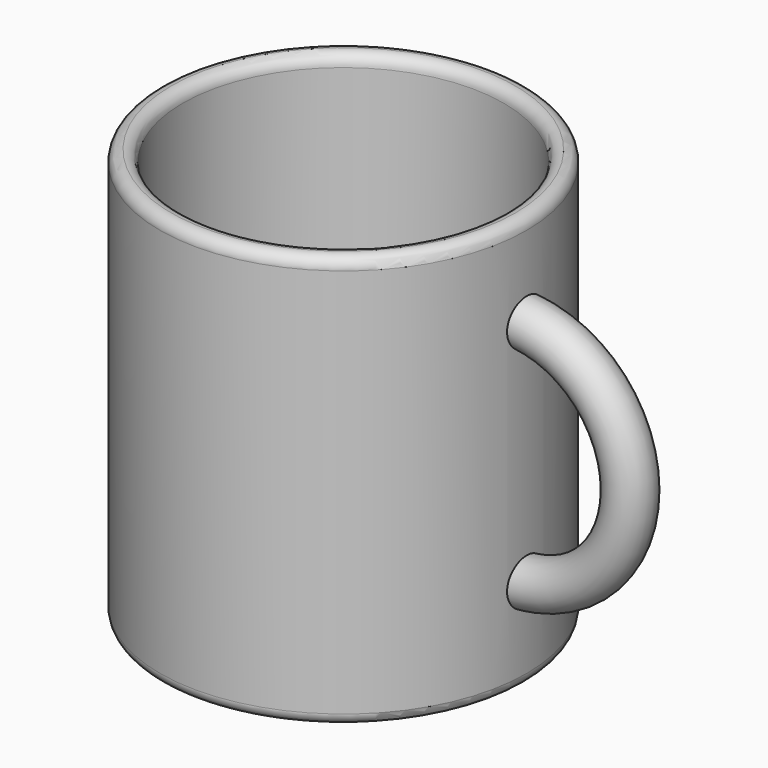
from build123d import *

# Parameters (mm, degrees)
F0_R         = 40
F1_DEPTH     = 90
F2_T         = -5
F4_R         = 5
F5_ANGLE     = 180
F6_R         = 2.49999
F7_TEXT_SIZE = 17.4750366973
F8_DEPTH     = 2.5


# Not quite as in the source:
# - a fillet or chamfer is up to 0.001 mm smaller than in the source, because OpenCascade refuses the exact size
# - Text() gives the source's letters only with a copy of the font that has no kerning and outlines rounded to 1/6400 em; it was checked with that copy


with BuildPart() as f1:
    # F0 (on Top) → F1 (new body)
    with BuildSketch(Plane.XY):
        Circle(F0_R)
    extrude(amount=F1_DEPTH)

    # F2
    f2_openings = [f1.faces().sort_by_distance(p)[0] for p in [
        (0, 0, 90),
    ]]
    offset(amount=F2_T, openings=f2_openings)

    # F4 (on offset) → F5 (revolve)
    with BuildSketch(Plane.YZ.offset(37.5)):
        with Locations((0, 70)):
            Circle(F4_R)
    revolve(axis=Axis((37.5, 15.199537389, 45), (0, 1, 0)), revolution_arc=F5_ANGLE)

    # F6 (radius 2.5 in the source; OpenCascade refuses exactly that, so slightly less here)
    f6_edges = [f1.edges().sort_by_distance(p)[0] for p in [
        (-40, 0, 90),
        (-35, 0, 90),
        (-40, 0, 0),
    ]]
    fillet(f6_edges, radius=F6_R)

    # F7 (on face) → F8 (cut)
    with BuildSketch(Plane(origin=(0, 0, 0), x_dir=(1, 0, 0), z_dir=(0, 0, -1))):
        with Locations((-37.1004994477, -5.4592069689)):
            Text('TOMBE2', F7_TEXT_SIZE, font='Open Sans', font_style=FontStyle.BOLD, text_align=(TextAlign.LEFT, TextAlign.BOTTOM))
    extrude(amount=-F8_DEPTH, mode=Mode.SUBTRACT)


solid = f1.part
